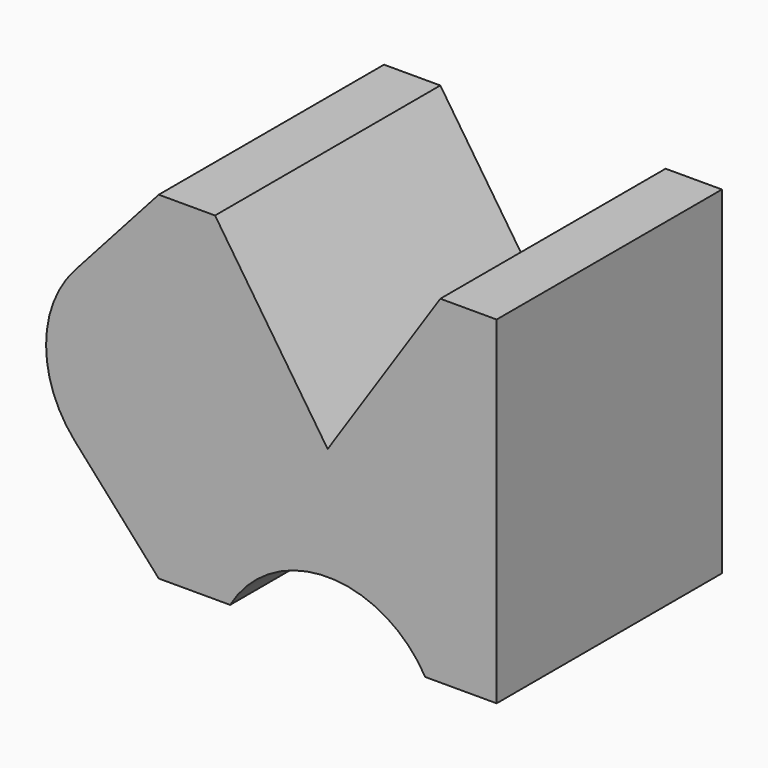
from build123d import *

# Parameters (mm, degrees)
F1_DEPTH = 25
F2_DEPTH = 25


# Not quite as in the source:
# - a feature of the source that left no trace in its solid (it failed there, or was rolled back) is left out


with BuildPart() as f1:
    # F0 (on Front) → F1 (new body)
    with BuildSketch(Plane.XZ):
        with BuildLine():
            Line((20, 30), (0, 0))
            Line((0, 0), (-20, 30))
            Line((-20, 30), (-30, 30))
            Line((-30, 30), (-44.90711985, 13.3333333333))
            ThreePointArc((-44.90711985, 13.3333333333), (-50, 0), (-44.90711985, -13.3333333333))
            Line((-44.90711985, -13.3333333333), (-30, -30))
            Line((-30, -30), (-17.3205080757, -30))
            ThreePointArc((-17.3205080757, -30), (0, -20), (17.3205080757, -30))
            Line((17.3205080757, -30), (30, -30))
            Line((30, -30), (30, 30))
            Line((30, 30), (20, 30))
        make_face()
    extrude(amount=F1_DEPTH)

    # F2 (add): a face of the model
    f2_faces = [f1.faces().sort_by_distance(p)[0] for p in [
        (-8.0009938, -25, -1.613641283),
    ]]
    extrude(f2_faces, amount=F2_DEPTH)


solid = f1.part
